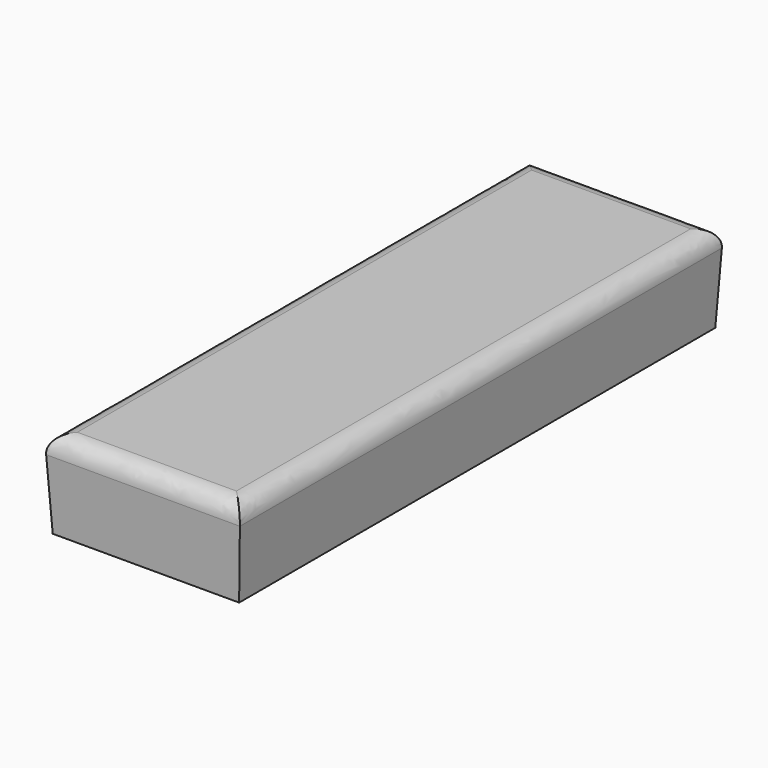
from build123d import *

# Parameters (mm, degrees)
F0_W     = 53.6705106497
F0_H     = 171.3497787714
F3_DEPTH = 25.4
F3_TAPER = -3
F5_R     = 5


# Not quite as in the source:
# - the program builds the solid bodies; features that only make, move or delete a surface that nothing else refers to are left out


with BuildPart() as f3:
    # F0 (on Top) → F3 (new body)
    with BuildSketch(Plane.XY):
        with Locations((26.8352553248, 85.6748893857)):
            Rectangle(F0_W, F0_H)
    extrude(amount=F3_DEPTH, taper=F3_TAPER)

    # F5
    f5_edges = [f3.edges().sort_by_distance(p)[0] for p in [
        (-1.331158, 85.674889, 25.4),
        (26.835255, -1.331158, 25.4),
        (55.001668, 85.674889, 25.4),
        (26.835255, 172.680936, 25.4),
    ]]
    fillet(f5_edges, radius=F5_R)


solid = f3.part
